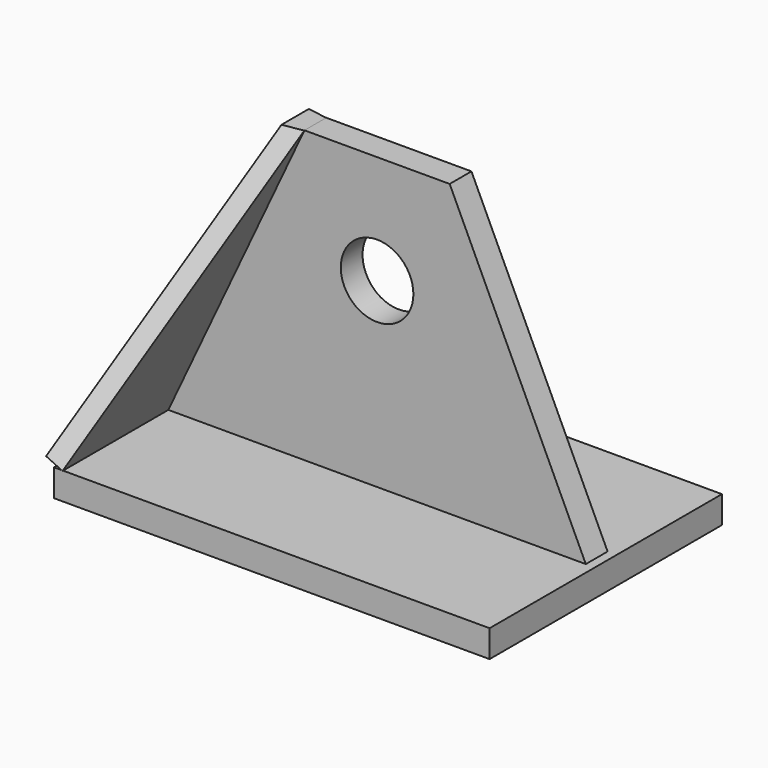
from build123d import *

# Parameters (mm, degrees)
F0_R        = 12.7
F1_DEPTH    = 4.7625
F2_W        = 152.4
F2_H        = 101.6
F3_DEPTH    = 9.525
F5_DEPTH    = 6.35
F6_T1_DEPTH = 43.3965999996


# Not quite as in the source:
# - a fillet or chamfer that OpenCascade refuses, or shapes differently, is made with other operations: its cross-section is extruded or revolved along the edge and cut away or added


with BuildPart() as f1:
    # F0 (on Front) → F1 (new body, symmetric)
    with BuildSketch(Plane.XZ):
        Polygon((-25.4, 101.6), (-73.025, 0), (73.025, 0), (25.4, 101.6), align=None)
        with Locations((0, 63.5)):
            Circle(F0_R, mode=Mode.SUBTRACT)
    extrude(amount=F1_DEPTH, both=True)


with BuildPart() as f3:
    # F2 (on face) → F3 (new body)
    with BuildSketch(Plane(origin=(0, 0, 0), x_dir=(1, 0, 0), z_dir=(0, 0, -1))):
        Rectangle(F2_W, F2_H)
    extrude(amount=F3_DEPTH)


with BuildPart() as f5:
    # F4 (on face) → F5 (new body)
    with BuildSketch(Plane(origin=(-59.8699759808, 0, 28.064051241), x_dir=(0, -1, 0), z_dir=(-0.905458936, 0, 0.4244338762))):
        Polygon((4.7625, 81.2140074372), (-4.7625, 81.2140074372), (-50.6641343236, -30.9942838117), (51.0465875268, -30.9942838117), align=None)
    extrude(amount=F5_DEPTH)

    # F6: chamfer of 3.048 x 6.5364570937 on 1 edges, made by hand

    # F6_s2 → F6_t1 (cut)
    with BuildSketch(Plane.XZ.offset(-21.6982999998)):
        Polygon((-25.2311707583, 101.520861293), (-32.4433386981, 101.5353162773), (-31.1496642433, 104.2951551141), align=None)
    extrude(amount=F6_T1_DEPTH, mode=Mode.SUBTRACT)


solid = Compound([f1.part, f3.part, f5.part])
